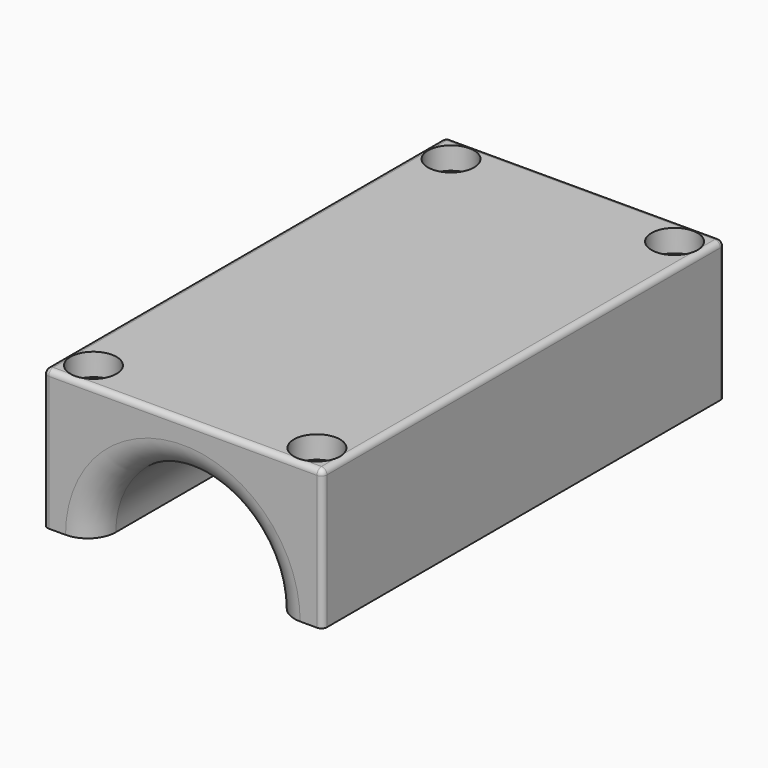
from build123d import *

# Parameters (mm, degrees)
F1_DEPTH       = 90
F3_D           = 4.4
F3_CBORE_D     = 8.25
F3_CBORE_DEPTH = 4
F4_R           = 5
F5_T1_DEPTH    = 88
F5_T3_DEPTH    = 26.5
F5_T5_DEPTH    = 48
F5_S9_W        = 1
F5_S9_H        = 1
F5_T10_DEPTH   = 1
F5_S15_W       = 1
F5_S15_H       = 1
F5_T16_DEPTH   = 1
F5_S21_W       = 1
F5_S21_H       = 1
F5_T22_DEPTH   = 1
F5_S27_W       = 1
F5_S27_H       = 1
F5_T28_DEPTH   = 1


# Not quite as in the source:
# - a fillet or chamfer that OpenCascade refuses, or shapes differently, is made with other operations: its cross-section is extruded or revolved along the edge and cut away or added


with BuildPart() as f1:
    # F0 (on Front) → F1 (new body)
    with BuildSketch(Plane.XZ):
        with BuildLine():
            Line((25, 0), (25, 25))
            Line((25, 25), (-25, 25))
            Line((-25, 25), (-25, 0))
            Line((-25, 0), (-16, 0))
            ThreePointArc((-16, 0), (0, 16), (16, 0))
            Line((16, 0), (25, 0))
        make_face()
    extrude(amount=F1_DEPTH)

    # F3 (through all)
    with Locations(Plane.XY.offset(25)):
        with Locations((-20, -85), (-20, -5), (20, -5), (20, -85)):
            CounterBoreHole(F3_D / 2, F3_CBORE_D / 2, F3_CBORE_DEPTH)

    # F4
    f4_edges = [f1.edges().sort_by_distance(p)[0] for p in [
        (0, -90, 16),
    ]]
    fillet(f4_edges, radius=F4_R)

    # F5: fillet of radius 1 on 8 edges, made by hand

    # F5_s2 → F5_t1 (cut)
    with BuildSketch(Plane.XZ.offset(1)):
        with BuildLine():
            ThreePointArc((25, 24), (24.7071067812, 24.7071067812), (24, 25))
            Line((24, 25), (25, 25))
            Line((25, 25), (25, 24))
        make_face()
        with BuildLine():
            ThreePointArc((-24, 25), (-24.7071067812, 24.7071067812), (-25, 24))
            Line((-25, 24), (-25, 25))
            Line((-25, 25), (-24, 25))
        make_face()
    extrude(amount=F5_T1_DEPTH, mode=Mode.SUBTRACT)

    # F5_s4 → F5_t3 (cut)
    with BuildSketch(Plane.XY.offset(-2.5)):
        with BuildLine():
            ThreePointArc((24, -90), (24.7071067812, -89.7071067812), (25, -89))
            Line((25, -89), (25, -90))
            Line((25, -90), (24, -90))
        make_face()
        with BuildLine():
            ThreePointArc((24, 0), (24.7071067812, -0.2928932188), (25, -1))
            Line((25, -1), (25, 0))
            Line((25, 0), (24, 0))
        make_face()
        with BuildLine():
            ThreePointArc((-24, 0), (-24.7071067812, -0.2928932188), (-25, -1))
            Line((-25, -1), (-25, 0))
            Line((-25, 0), (-24, 0))
        make_face()
        with BuildLine():
            ThreePointArc((-24, -90), (-24.7071067812, -89.7071067812), (-25, -89))
            Line((-25, -89), (-25, -90))
            Line((-25, -90), (-24, -90))
        make_face()
    extrude(amount=F5_T3_DEPTH, mode=Mode.SUBTRACT)

    # F5_s6 → F5_t5 (cut)
    with BuildSketch(Plane.YZ.offset(-24)):
        with BuildLine():
            ThreePointArc((0, 24), (-0.2928932188, 24.7071067812), (-1, 25))
            Line((-1, 25), (0, 25))
            Line((0, 25), (0, 24))
        make_face()
        with BuildLine():
            ThreePointArc((-90, 24), (-89.7071067812, 24.7071067812), (-89, 25))
            Line((-89, 25), (-90, 25))
            Line((-90, 25), (-90, 24))
        make_face()
    extrude(amount=F5_T5_DEPTH, mode=Mode.SUBTRACT)


with BuildPart() as f5_tool8:
    # F5_s9 → F5_t10 (new body)
    with BuildSketch(Plane.XY.offset(24)):
        with Locations((24.5, -0.5)):
            Rectangle(F5_S9_W, F5_S9_H)
    extrude(amount=F5_T10_DEPTH)

    # F5_s11 → F5_t12 (revolve, cut)
    with BuildSketch(Plane(origin=(24, -1, 24), x_dir=(-0.7071067812, -0.7071067812, 0), z_dir=(-0.7071067812, 0.7071067812, 0))):
        with BuildLine():
            ThreePointArc((0, -1), (1, 0), (0, 1))
            Line((0, 1), (0, -1))
        make_face()
    revolve(axis=Axis((24, -1, 24), (0, 0, 1)), mode=Mode.SUBTRACT)


with BuildPart() as f1_1:
    add(f1.part)

    # F5_t7: cut F5_tool8
    add(f5_tool8.part, mode=Mode.SUBTRACT)


with BuildPart() as f5_tool14:
    # F5_s15 → F5_t16 (new body)
    with BuildSketch(Plane.XY.offset(24)):
        with Locations((24.5, -89.5)):
            Rectangle(F5_S15_W, F5_S15_H)
    extrude(amount=F5_T16_DEPTH)

    # F5_s17 → F5_t18 (revolve, cut)
    with BuildSketch(Plane(origin=(24, -89, 24), x_dir=(-0.7071067812, 0.7071067812, 0), z_dir=(0.7071067812, 0.7071067812, 0))):
        with BuildLine():
            ThreePointArc((0, -1), (1, 0), (0, 1))
            Line((0, 1), (0, -1))
        make_face()
    revolve(axis=Axis((24, -89, 24), (0, 0, 1)), mode=Mode.SUBTRACT)


with BuildPart() as f1_2:
    add(f1_1.part)

    # F5_t13: cut F5_tool14
    add(f5_tool14.part, mode=Mode.SUBTRACT)


with BuildPart() as f5_tool20:
    # F5_s21 → F5_t22 (new body)
    with BuildSketch(Plane.XY.offset(24)):
        with Locations((-24.5, -0.5)):
            Rectangle(F5_S21_W, F5_S21_H)
    extrude(amount=F5_T22_DEPTH)

    # F5_s23 → F5_t24 (revolve, cut)
    with BuildSketch(Plane(origin=(-24, -1, 24), x_dir=(0.7071067812, -0.7071067812, 0), z_dir=(-0.7071067812, -0.7071067812, 0))):
        with BuildLine():
            ThreePointArc((0, -1), (1, 0), (0, 1))
            Line((0, 1), (0, -1))
        make_face()
    revolve(axis=Axis((-24, -1, 24), (0, 0, 1)), mode=Mode.SUBTRACT)


with BuildPart() as f1_3:
    add(f1_2.part)

    # F5_t19: cut F5_tool20
    add(f5_tool20.part, mode=Mode.SUBTRACT)


with BuildPart() as f5_tool26:
    # F5_s27 → F5_t28 (new body)
    with BuildSketch(Plane.XY.offset(24)):
        with Locations((-24.5, -89.5)):
            Rectangle(F5_S27_W, F5_S27_H)
    extrude(amount=F5_T28_DEPTH)

    # F5_s29 → F5_t30 (revolve, cut)
    with BuildSketch(Plane(origin=(-24, -89, 24), x_dir=(0.7071067812, 0.7071067812, 0), z_dir=(0.7071067812, -0.7071067812, 0))):
        with BuildLine():
            ThreePointArc((0, -1), (1, 0), (0, 1))
            Line((0, 1), (0, -1))
        make_face()
    revolve(axis=Axis((-24, -89, 24), (0, 0, 1)), mode=Mode.SUBTRACT)


with BuildPart() as f1_4:
    add(f1_3.part)

    # F5_t25: cut F5_tool26
    add(f5_tool26.part, mode=Mode.SUBTRACT)


solid = f1_4.part
